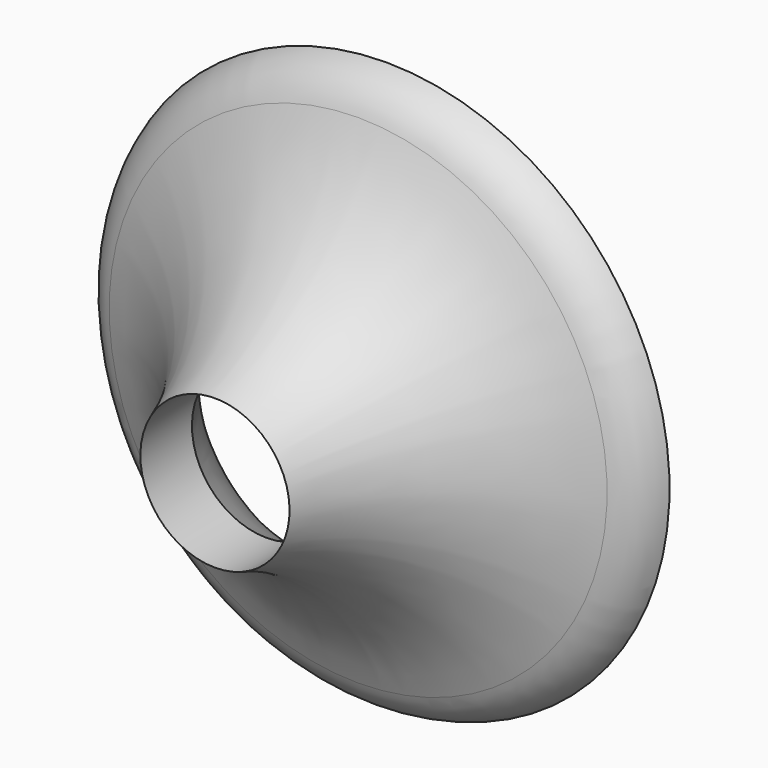
from build123d import *


# Not quite as in the source:
# - a fillet or chamfer that OpenCascade refuses, or shapes differently, is made with other operations: its cross-section is extruded or revolved along the edge and cut away or added


with BuildPart() as f1:
    # F0 (on Right) → F1 (revolve)
    with BuildSketch(Plane.YZ):
        with BuildLine():
            Line((-2.2878659654, -26.3821920429), (0.1111427558, -26.3821920429))
            ThreePointArc((0.1111427558, -26.3821920429), (-4.5151946669, -15.0073463307), (-13.8172382977, -6.9909819916))
            Line((-13.8172382977, -6.9909819916), (-19.8118997502, -6.9909819916))
            ThreePointArc((-19.8118997502, -6.9909819916), (-8.4327201707, -14.3214304732), (-2.2878659654, -26.3821920429))
        make_face()
    revolve(axis=Axis((0, -9.8503784972, -0.0567880845), (0, -1, 0)))

    # F2: fillet of radius 5.08 on 1 edges, made by hand

    # F2_s1 → F2_t2 (revolve, cut)
    with BuildSketch(Plane.YZ):
        with BuildLine():
            ThreePointArc((0.1111427558, -26.3821920429), (-1.9081947571, -25.1822984596), (-3.171877995, -23.2022547035))
            ThreePointArc((-3.171877995, -23.2022547035), (-2.6793038851, -24.7781656105), (-2.2878659654, -26.3821920429))
            Line((-2.2878659654, -26.3821920429), (0.1111427558, -26.3821920429))
        make_face()
    revolve(axis=Axis((0, -2.2878659654, -0.0567880845), (0, -1, 0)), mode=Mode.SUBTRACT)


solid = f1.part
